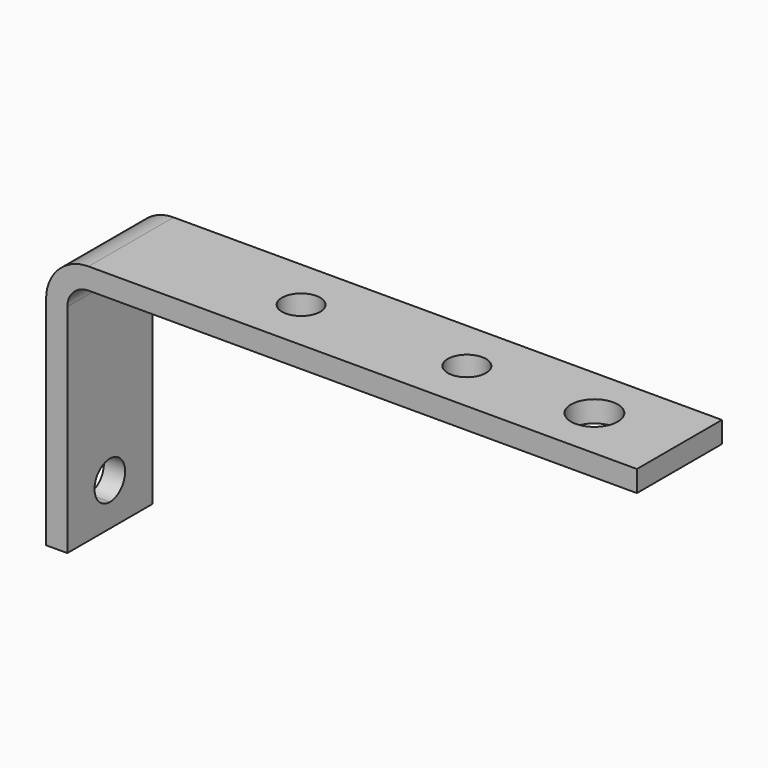
from build123d import *

# Parameters (mm, degrees)
F1_DEPTH = 25
F2_R     = 5.5
F2_R_2   = 4.5
F3_DEPTH = 5
F4_DEPTH = 5
F6_DEPTH = 5


# Not quite as in the source:
# - ends of sketch curves that miss each other by under 0.0002 mm in the source are joined


with BuildPart() as f1:
    # F0 (on Front) → F1 (new body)
    with BuildSketch(Plane.XZ):
        with BuildLine():
            Line((134, 0), (134, 5))
            Line((134, 5), (5, 5))
            ThreePointArc((5, 5), (2.4118095455, 4.6592580848), (0, 3.6602538402))
            Line((0, 3.6602538402), (0, 0))
            Line((0, 0), (5, 0))
            Line((5, 0), (134, 0))
        make_face()
        with BuildLine():
            Line((0, 0), (0, 3.6602538402))
            ThreePointArc((0, 3.6602538402), (-3.6602539143, -1.284e-07), (-4.9999998289, -5))
            Line((-4.9999998289, -5), (-5, -56))
            Line((-5, -56), (0, -56))
            Line((0, -56), (0, -5))
            Line((0, -5), (0, 0))
        make_face()
        with BuildLine():
            ThreePointArc((0, -5), (1.4644660941, -1.4644660941), (5, 0))
            Line((5, 0), (0, 0))
            Line((0, 0), (0, -5))
        make_face()
    extrude(amount=-F1_DEPTH)

    # F2 (on face) → F3 (cut)
    with BuildSketch(Plane.XY.offset(5)):
        with Locations((114, 12.5)):
            Circle(F2_R)
        with Locations((84, 12.5)):
            Circle(F2_R_2)
        with Locations((45, 12.5)):
            Circle(F2_R_2)
    extrude(amount=-F3_DEPTH, mode=Mode.SUBTRACT)

    # F2 (on face) → F4 (cut)
    with BuildSketch(Plane.XY.offset(5)):
        with Locations((114, 12.5)):
            Circle(F2_R)
        with Locations((84, 12.5)):
            Circle(F2_R_2)
        with Locations((45, 12.5)):
            Circle(F2_R_2)
    extrude(amount=-F4_DEPTH, mode=Mode.SUBTRACT)

    # F5 (on face) → F6 (cut)
    with BuildSketch(Plane(origin=(-5, 0, 0), x_dir=(0, -1, 0), z_dir=(-1, 0, 0))):
        with BuildLine():
            ThreePointArc((-12.5, -50.5), (-9.3180194847, -49.1819805153), (-8, -46))
            ThreePointArc((-8, -46), (-15.6819805153, -42.8180194847), (-12.5, -50.5))
        make_face()
    extrude(amount=-F6_DEPTH, mode=Mode.SUBTRACT)


solid = f1.part
